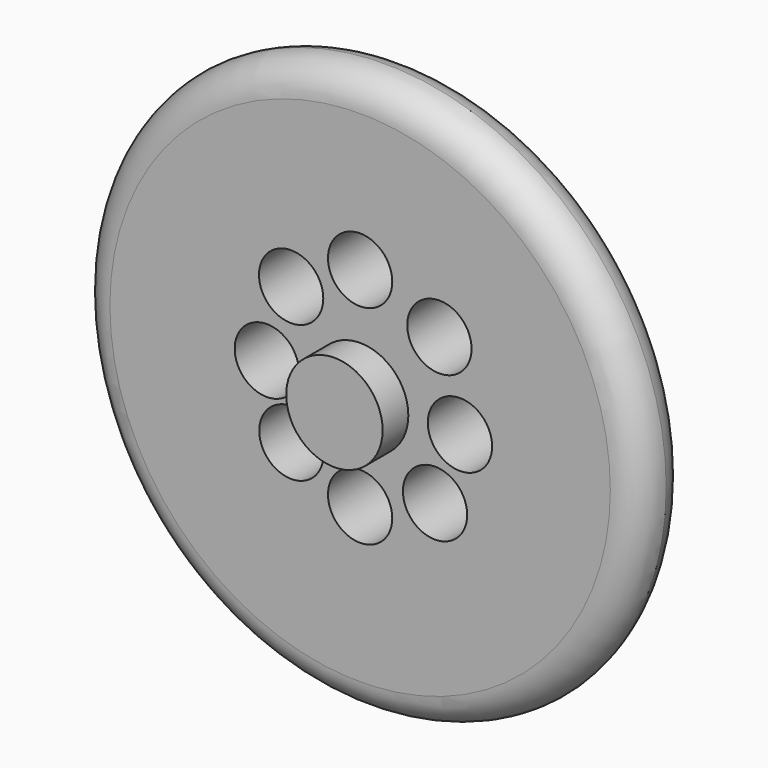
from build123d import *

# Parameters (mm, degrees)
F0_R     = 3
F1_DEPTH = 11
F3_DEPTH = 2
F2_R     = 17.5
F4_DEPTH = 4
F5_R     = 1.9313708499
F7_R     = 2
F8_DEPTH = 6.5


# Not quite as in the source:
# - a fillet or chamfer that OpenCascade refuses, or shapes differently, is made with other operations: its cross-section is extruded or revolved along the edge and cut away or added


with BuildPart() as f1:
    # F0 (on Front) → F1 (new body)
    with BuildSketch(Plane.XZ):
        Circle(F0_R)
    extrude(amount=-F1_DEPTH)

    # F0 (on Front) → F3 (join)
    with BuildSketch(Plane.XZ):
        Circle(F0_R)
    extrude(amount=F3_DEPTH)

    # F2 (on Front) → F4 (join)
    with BuildSketch(Plane.XZ):
        Circle(F2_R)
    extrude(amount=-F4_DEPTH)

    # F5
    f5_edges = [f1.edges().sort_by_distance(p)[0] for p in [
        (-17.5, 0, 0),
    ]]
    fillet(f5_edges, radius=F5_R)

    # F6: fillet of radius 2.4142135624 on 1 edges, made by hand

    # F6_s1 → F6_t2 (revolve, cut)
    with BuildSketch(Plane.XY):
        with BuildLine():
            ThreePointArc((17.5, 1.9313708499), (16.6908565976, 3.4109907686), (15.1106489294, 4))
            Line((15.1106489294, 4), (15.1106489294, 4.0482842712))
            Line((15.1106489294, 4.0482842712), (17.5, 4.0482842712))
            Line((17.5, 4.0482842712), (17.5482842712, 4))
            ThreePointArc((17.5482842712, 4), (17.5482842712, 2.9656854249), (17.5477870214, 1.9382825381))
            Line((17.5477870214, 1.9382825381), (17.5, 1.9313708499))
        make_face()
    revolve(axis=Axis((0, 4, 0), (0, -1, 0)), mode=Mode.SUBTRACT)

    # F7 (on face) → F8 (cut)
    with BuildSketch(Plane.XZ):
        with Locations((0, -5.9548519258)):
            Circle(F7_R)
        with Locations((6.2130242586, 0)):
            Circle(F7_R)
        with Locations((4.9334257519, 4.926879719)):
            Circle(F7_R)
        with Locations((0, 7)):
            Circle(F7_R)
        with Locations((4.6638702957, -4.2616006167)):
            Circle(F7_R)
        with Locations((-4.2754073071, -3.8503200899)):
            Circle(F7_R)
        with Locations((-4.2925996605, 4.681295439)):
            Circle(F7_R)
        with Locations((-5.8032550169, 0.1451130412)):
            Circle(F7_R)
    extrude(amount=-F8_DEPTH, mode=Mode.SUBTRACT)


solid = f1.part
